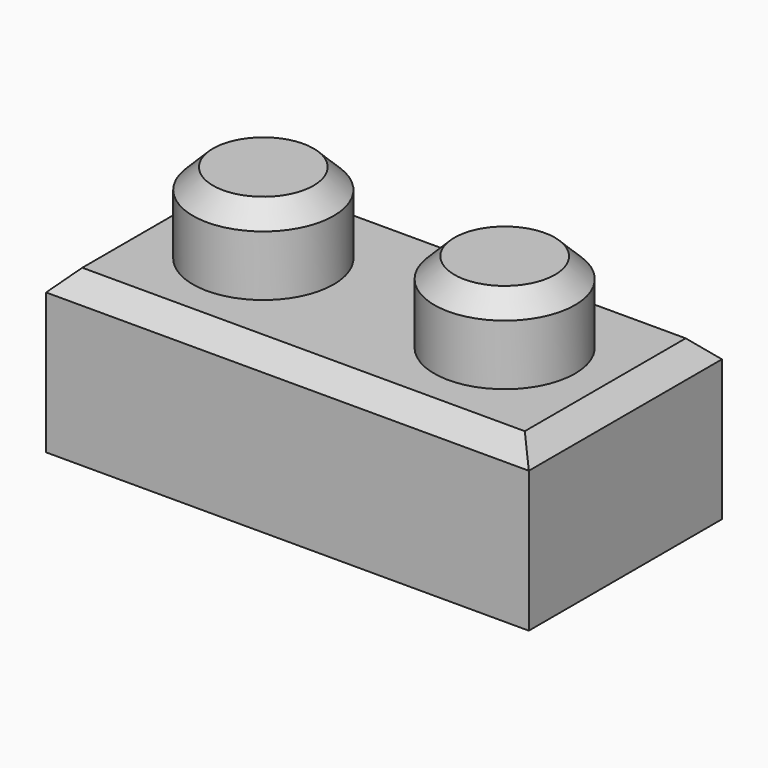
from build123d import *

# Parameters (mm, degrees)
F0_W     = 76.2
F0_H     = 38.1
F1_DEPTH = 25.4
F2_R     = 11.1125
F3_DEPTH = 12.7
F4_SIZE  = 3.175
F5_T     = 7.9375


# Not quite as in the source:
# - a shell that OpenCascade refuses in one call is made with other operations: the cavity is built on its own and cut out


with BuildPart() as f1:
    # F0 (on Top) → F1 (new body)
    with BuildSketch(Plane.XY):
        with Locations((25.6543946505, -9.0019332737)):
            Rectangle(F0_W, F0_H)
    extrude(amount=F1_DEPTH)

    # F2 (on face) → F3 (join)
    with BuildSketch(Plane.XY.offset(25.4)):
        with Locations((6.6043946505, -9.0019332737)):
            Circle(F2_R)
        with Locations((44.7043946505, -9.0019332737)):
            Circle(F2_R)
    extrude(amount=F3_DEPTH)

    # F4
    f4_edges = [f1.edges().sort_by_distance(p)[0] for p in [
        (-4.508105, -9.001933, 38.1),
        (33.591895, -9.001933, 38.1),
        (-12.445605, -9.001933, 25.4),
        (25.654395, 10.048067, 25.4),
        (25.654395, -28.051933, 25.4),
        (63.754395, -9.001933, 25.4),
    ]]
    chamfer(f4_edges, length=F4_SIZE)

    # F5: shell of thickness 7.9375, made by hand


with BuildPart() as f5_core1:
    # F5_t2: copy of F1
    add(f1.part)

    # the walls: a layer under each face that stays
    f5_faces = [f5_core1.faces().sort_by_distance(p)[0] for p in [
        (25.6543946505, -28.0519332737, 11.1125),
        (-12.4456053495, -9.0019332737, 11.1125),
        (25.6543946505, -26.4644332737, 23.8125),
        (63.7543946505, -9.0019332737, 11.1125),
        (25.6543946505, 10.0480667263, 11.1125),
        (-10.8581053495, -9.0019332737, 23.8125),
        (25.6543946505, -9.0019332737, 25.4),
        (62.1668946505, -9.0019332737, 23.8125),
        (25.6543946505, 8.4605667263, 23.8125),
        (33.5918946505, -9.0019332737, 30.1625),
        (-4.5081053495, -9.0019332737, 30.1625),
        (35.1793946505, -9.0019332737, 36.5125),
        (-2.9206053495, -9.0019332737, 36.5125),
        (44.7043946505, -9.0019332737, 38.1),
        (6.6043946505, -9.0019332737, 38.1),
    ]]
    thicken(f5_faces, amount=-F5_T, mode=Mode.SUBTRACT)

    # F5_s3 → F5_t4 (revolve, cut)
    with BuildSketch(Plane.XZ.offset(9.0019332737)):
        Polygon((55.8962696505, 25.479375), (55.8168946505, 17.4625), (47.8793946505, 17.4625), (47.8793946505, 25.4), align=None)
    revolve(axis=Axis((44.7043946505, -9.0019332737, 25.4), (0, 0, 1)), mode=Mode.SUBTRACT)

    # F5_s5 → F5_t6 (revolve, cut)
    with BuildSketch(Plane.XZ.offset(9.0019332737)):
        Polygon((17.7962696505, 25.479375), (17.7168946505, 17.4625), (9.7793946505, 17.4625), (9.7793946505, 25.4), align=None)
    revolve(axis=Axis((6.6043946505, -9.0019332737, 25.4), (0, 0, 1)), mode=Mode.SUBTRACT)


with BuildPart() as f1_1:
    add(f1.part)

    # what is left inside the walls is the cavity
    f5_cavity = [f5_core1.part.solids().sort_by_distance(p)[0] for p in [
        (25.654395, -12.7061, 0.079375),
    ]]
    add(f5_cavity, mode=Mode.SUBTRACT)


solid = f1_1.part
